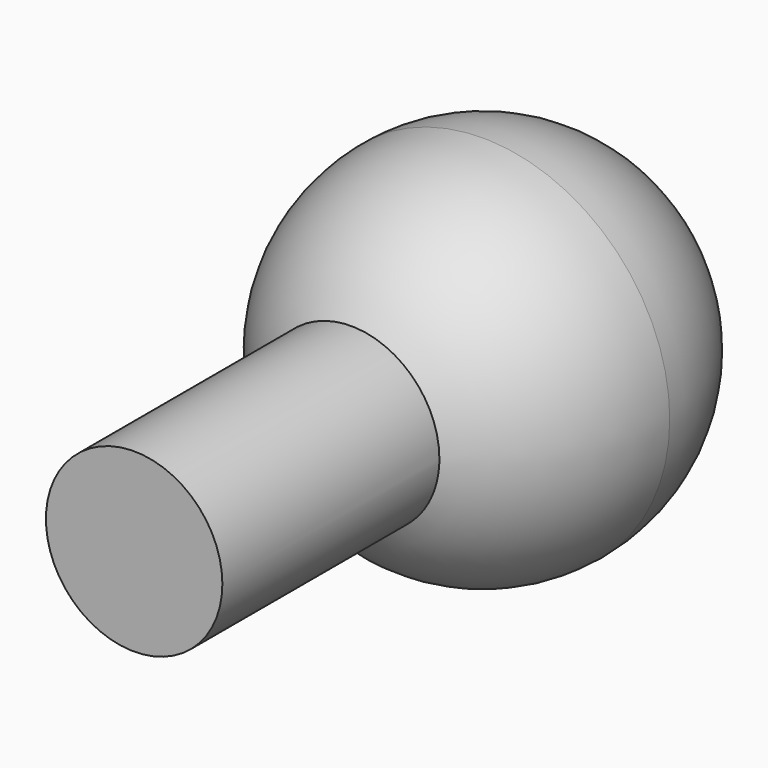
from build123d import *

# Parameters (mm, degrees)
F2_R     = 4.25
F3_DEPTH = 21


with BuildPart() as f1:
    # F0 (on Top) → F1 (revolve)
    with BuildSketch(Plane.XY):
        with BuildLine():
            ThreePointArc((0, -9), (6.3639610307, -6.3639610307), (9, 0))
            ThreePointArc((9, 0), (6.3639610307, 6.3639610307), (0, 9))
            Line((0, 9), (0, 0))
            Line((0, 0), (0, -9))
        make_face()
    revolve(axis=Axis((0, 0, 0), (0, -1, 0)))

    # F2 (on Front) → F3 (join)
    with BuildSketch(Plane.XZ):
        Circle(F2_R)
    extrude(amount=F3_DEPTH)


solid = f1.part
